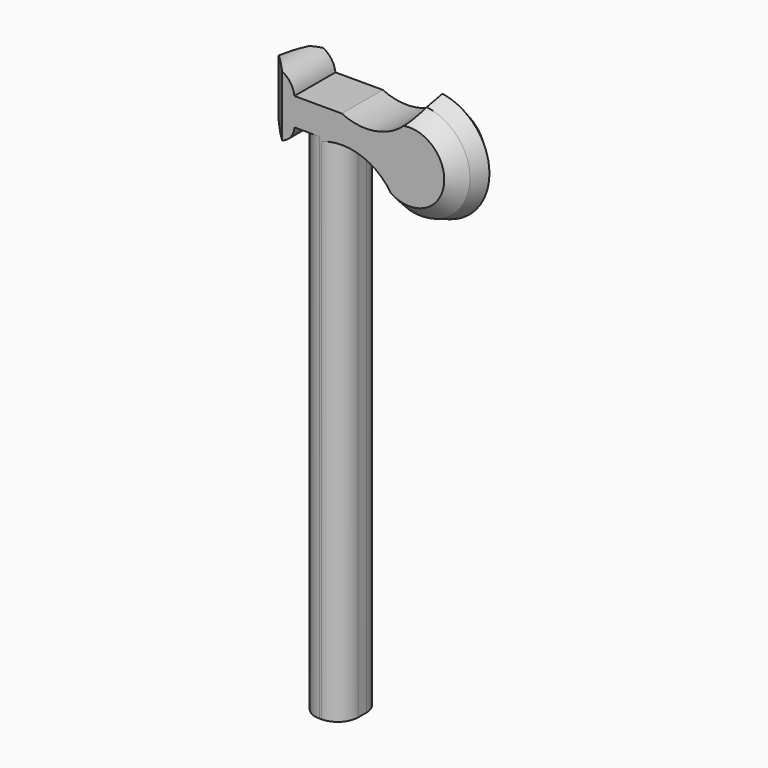
from build123d import *

# Parameters (mm, degrees)
F0_W        = 10.6210811783
F0_H        = 127
F1_DEPTH    = 6.35
F2_DEPTH    = 6.35
F3_SIZE     = 5.334
F4_T2_ANGLE = 234.6452810907
F5_SIZE     = 5.588
F6_T1_DEPTH = 37.3754237446
F7_R        = 5.08
F8_R        = 5.08


# Not quite as in the source:
# - a fillet or chamfer that OpenCascade refuses, or shapes differently, is made with other operations: its cross-section is extruded or revolved along the edge and cut away or added
# - a feature names something its author has since deleted; it is built from what else it names


with BuildPart() as f1:
    # F0 (on Front) → F1 (new body)
    with BuildSketch(Plane.XZ):
        with BuildLine():
            ThreePointArc((-31.2650664442, 63.9850506011), (-26.8698078998, 60.1482815757), (-22.6583778858, 64.185972929))
            Line((-22.6583778858, 64.185972929), (-21.5300321579, 64.185972929))
            Line((-21.5300321579, 64.185972929), (-10.9089509796, 64.185972929))
            ThreePointArc((-10.9089509796, 64.185972929), (-1.1488196144, 60.4281603773), (3.5711703362, 51.0952608115))
            ThreePointArc((3.5711703362, 51.0952608115), (19.6335156732, 62.5824206191), (8.0880673261, 78.602920007))
            ThreePointArc((8.0880673261, 78.602920007), (0.2340476898, 70.6911078158), (-10.9089509796, 71.0316621421))
            Line((-10.9089509796, 71.0316621421), (-22.6583778858, 71.0316621421))
            ThreePointArc((-22.6583778858, 71.0316621421), (-25.8366796537, 75.4537471146), (-31.2650664442, 75.0189431538))
            Line((-31.2650664442, 75.0189431538), (-31.2650664442, 63.9850506011))
        make_face()
        with Locations((-16.2194915688, 0.685972929)):
            Rectangle(F0_W, F0_H)
    extrude(amount=F1_DEPTH)

    # F0 (on Front) → F2 (join)
    with BuildSketch(Plane.XZ):
        with BuildLine():
            ThreePointArc((-31.2650664442, 63.9850506011), (-26.8698078998, 60.1482815757), (-22.6583778858, 64.185972929))
            Line((-22.6583778858, 64.185972929), (-21.5300321579, 64.185972929))
            Line((-21.5300321579, 64.185972929), (-10.9089509796, 64.185972929))
            ThreePointArc((-10.9089509796, 64.185972929), (-1.1488196144, 60.4281603773), (3.5711703362, 51.0952608115))
            ThreePointArc((3.5711703362, 51.0952608115), (19.6335156732, 62.5824206191), (8.0880673261, 78.602920007))
            ThreePointArc((8.0880673261, 78.602920007), (0.2340476898, 70.6911078158), (-10.9089509796, 71.0316621421))
            Line((-10.9089509796, 71.0316621421), (-22.6583778858, 71.0316621421))
            ThreePointArc((-22.6583778858, 71.0316621421), (-25.8366796537, 75.4537471146), (-31.2650664442, 75.0189431538))
            Line((-31.2650664442, 75.0189431538), (-31.2650664442, 63.9850506011))
        make_face()
        with Locations((-16.2194915688, 0.685972929)):
            Rectangle(F0_W, F0_H)
    extrude(amount=-F2_DEPTH)

    # F3
    f3_edges = [f1.edges().sort_by_distance(p)[0] for p in [
        (19.633516, -6.35, 62.582421),
        (19.633516, 6.35, 62.582421),
    ]]
    chamfer(f3_edges, length=F3_SIZE)

    # F4: chamfer of 2.54 on 1 edges, made by hand

    # F4_s1 → F4_t2 (revolve, cut)
    with BuildSketch(Plane(origin=(-27.2674669531, 0, 20.2858371039), x_dir=(0, 1, 0), z_dir=(-0.8023210272, 0, 0.596892762))):
        Polygon((1.524, -41.5945799258), (-2.8120512242, -43.39063115), (-1.016, -41.5945799258), align=None)
    revolve(axis=Axis((5.8795952776, -1.016, 64.8408840236), (0, -1, 0)), revolution_arc=F4_T2_ANGLE, mode=Mode.SUBTRACT)

    # F5
    f5_edges = [f1.edges().sort_by_distance(p)[0] for p in [
        (-31.265066, 6.35, 69.501997),
        (-31.265066, -6.35, 69.501997),
    ]]
    chamfer(f5_edges, length=F5_SIZE)

    # F6: chamfer of 5.08 on 1 edges, made by hand

    # F6_s2 → F6_t1 (cut)
    with BuildSketch(Plane.XY.offset(50.8142850052)):
        Polygon((-31.2650664442, -4.318), (-27.6729639958, 4.3541024484), (-31.2650664442, 0.762), align=None)
    extrude(amount=F6_T1_DEPTH, mode=Mode.SUBTRACT)

    # F7
    f7_edges = [f1.edges().sort_by_distance(p)[0] for p in [
        (-10.908951, -6.35, 0.685973),
        (-10.908951, 6.35, 0.685973),
    ]]
    fillet(f7_edges, radius=F7_R)

    # F8
    f8_edges = [f1.edges().sort_by_distance(p)[0] for p in [
        (-21.530032, 6.35, 0.685973),
        (-21.530032, -6.35, 0.685973),
    ]]
    fillet(f8_edges, radius=F8_R)


solid = f1.part
